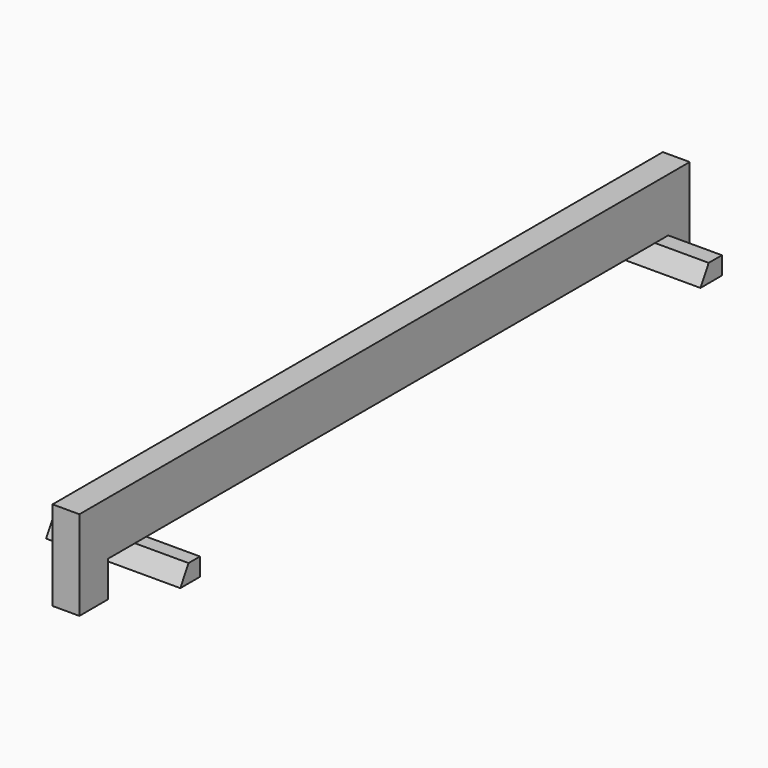
from build123d import *

# Parameters (mm, degrees)
F1_DEPTH  = 19.05
F3_DEPTH  = 38.1
F5_DEPTH  = 38.1
F7_DEPTH  = 19.05
F9_DEPTH  = 57.15
F10_DEPTH = 38.1
F11_W     = 19.05
F11_H     = 38.1
F12_DEPTH = 25.4
F13_W     = 19.05
F13_H     = 19.05
F13_H_2   = 6.35
F14_DEPTH = 25.4
F15_DEPTH = 38.1


# Not quite as in the source:
# - a feature names something its author has since deleted; it is built from what else it names


with BuildPart() as f1:
    # F0 (on Right) → F1 (new body)
    with BuildSketch(Plane.YZ):
        Polygon((-19.05, 0), (0, 0), (0, 50.8), (-477.8375, 50.8), (-477.8375, 12.7), (-11.7176515813, 12.7), align=None)
    extrude(amount=F1_DEPTH)

    # F2 (on face) → F3 (join)
    with BuildSketch(Plane.YZ.offset(19.05)):
        Polygon((0, 12.7), (-11.7176515813, 12.7), (-19.05, 0), (0, 0), align=None)
    extrude(amount=F3_DEPTH)

    # F4 (on face) → F5 (join)
    with BuildSketch(Plane(origin=(0, 0, 0), x_dir=(0, -1, 0), z_dir=(-1, 0, 0))):
        Polygon((19.05, 0), (11.7176515813, 12.7), (0, 12.7), (0, 0), align=None)
    extrude(amount=F5_DEPTH)

    # F6 (on face) → F7 (join)
    with BuildSketch(Plane(origin=(0, 0, 0), x_dir=(-1, 0, 0), z_dir=(0, 1, 0))):
        Polygon((0, 50.8), (-19.05, 50.8), (-19.05, 12.7), (-19.05, 0), (0, 0), (0, 12.7), align=None)
    extrude(amount=F7_DEPTH)

    # F8 (on face) → F9 (join)
    with BuildSketch(Plane.YZ.offset(19.05)):
        Polygon((-462.9448484187, 12.7), (-473.075, 12.7), (-480.4073484187, 0), (-462.9448484187, 0), align=None)
    extrude(amount=-F9_DEPTH)

    # F8 (on face) → F10 (join)
    with BuildSketch(Plane.YZ.offset(19.05)):
        Polygon((-462.9448484187, 12.7), (-473.075, 12.7), (-480.4073484187, 0), (-462.9448484187, 0), align=None)
    extrude(amount=F10_DEPTH)

    # F11 (on face) → F12 (join)
    with BuildSketch(Plane.XZ.offset(477.8375)):
        with Locations((9.525, 31.75)):
            Rectangle(F11_W, F11_H)
    extrude(amount=F12_DEPTH)

    # F13 (on face) → F14 (join)
    with BuildSketch(Plane(origin=(0, 0, 12.7), x_dir=(1, 0, 0), z_dir=(0, 0, -1))):
        with Locations((9.525, 512.7625)):
            Rectangle(F13_W, F13_H)
        with Locations((9.525, 500.0625)):
            Rectangle(F13_W, F13_H_2)
    extrude(amount=F14_DEPTH)

    # F15 (add, through all): a face of the model
    f15_faces = [f1.faces().sort_by_distance(p)[0] for p in [
        (9.525, -512.7625, 12.7),
    ]]
    extrude(f15_faces, amount=F15_DEPTH)


solid = f1.part
